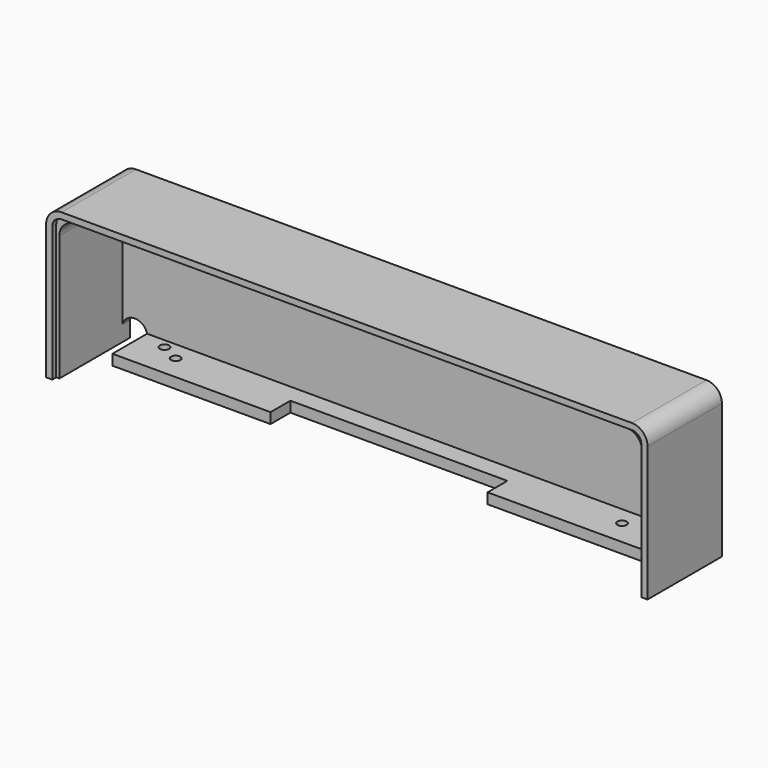
from build123d import *

# Parameters (mm, degrees)
F1_DEPTH = 30
F2_DEPTH = 28.4
F0_W     = 2.5
F0_H     = 3.4
F0_W_2   = 3
F0_W_3   = 7
F0_W_4   = 35.5
F0_W_5   = 70
F3_DEPTH = 17
F0_R     = 1.75
F4_DEPTH = 3
F6_DEPTH = 25
F7_R     = 1.5
F7_W     = 70
F7_H     = 13.8912867606
F8_DEPTH = 25


# Not quite as in the source:
# - ends of sketch curves that miss each other by under 0.0002 mm in the source are joined


with BuildPart() as f1:
    # F0 (on Front) → F1 (new body)
    with BuildSketch(Plane.XZ):
        with BuildLine():
            Line((-180.478038, -29.2658), (-180.478038, -72.7658))
            Line((-180.478038, -72.7658), (-178.478038, -72.7658))
            Line((-178.478038, -72.7658), (-178.478038, -29.2658))
            ThreePointArc((-178.478038, -29.2658), (-177.5993583436, -27.1444796564), (-175.478038, -26.2658))
            Line((-175.478038, -26.2658), (8.521962, -26.2658))
            ThreePointArc((8.521962, -26.2658), (10.6432823436, -27.1444796564), (11.521962, -29.2658))
            Line((11.521962, -29.2658), (11.521962, -71.1658))
            Line((11.521962, -71.1658), (11.521962, -72.7658))
            Line((11.521962, -72.7658), (13.521962, -72.7658))
            Line((13.521962, -72.7658), (13.521962, -29.2658))
            ThreePointArc((13.521962, -29.2658), (12.0574959059, -25.7302660941), (8.521962, -24.2658))
            Line((8.521962, -24.2658), (-175.478038, -24.2658))
            ThreePointArc((-175.478038, -24.2658), (-179.0135719059, -25.7302660941), (-180.478038, -29.2658))
        make_face()
    extrude(amount=F1_DEPTH)

    # F0 (on Front) → F2 (join)
    with BuildSketch(Plane.XZ):
        with BuildLine():
            Line((-178.478038, -29.2658), (-178.478038, -72.7658))
            Line((-178.478038, -72.7658), (-177.478038, -72.7658))
            Line((-177.478038, -72.7658), (-177.478038, -67.7658000352))
            Line((-177.478038, -67.7658000352), (-177.478038, -32.2658))
            ThreePointArc((-177.478038, -32.2658), (-176.0135719059, -28.7302660941), (-172.478038, -27.2658))
            Line((-172.478038, -27.2658), (5.521962, -27.2658))
            ThreePointArc((5.521962, -27.2658), (9.0574959059, -28.7302660941), (10.521962, -32.2658))
            Line((10.521962, -32.2658), (10.521962, -62.7658))
            Line((10.521962, -62.7658), (10.521962, -71.1658))
            Line((10.521962, -71.1658), (11.521962, -71.1658))
            Line((11.521962, -71.1658), (11.521962, -29.2658))
            ThreePointArc((11.521962, -29.2658), (10.6432823436, -27.1444796564), (8.521962, -26.2658))
            Line((8.521962, -26.2658), (-175.478038, -26.2658))
            ThreePointArc((-175.478038, -26.2658), (-177.5993583436, -27.1444796564), (-178.478038, -29.2658))
        make_face()
    extrude(amount=F2_DEPTH)

    # F0 (on Front) → F3 (join)
    with BuildSketch(Plane.XZ):
        with Locations((-168.228038, -69.4658)):
            Rectangle(F0_W, F0_H)
        with Locations((-165.478038, -69.4658)):
            Rectangle(F0_W_2, F0_H)
        with Locations((-160.478038, -69.4658)):
            Rectangle(F0_W_3, F0_H)
        with Locations((-155.478038, -69.4658)):
            Rectangle(F0_W_2, F0_H)
        with Locations((-136.228038, -69.4658)):
            Rectangle(F0_W_4, F0_H)
        with Locations((-83.478038, -69.4658)):
            Rectangle(F0_W_5, F0_H)
        with Locations((-30.728038, -69.4658)):
            Rectangle(F0_W_4, F0_H)
        with Locations((-11.478038, -69.4658)):
            Rectangle(F0_W_2, F0_H)
        with Locations((-6.478038, -69.4658)):
            Rectangle(F0_W_3, F0_H)
        with Locations((-1.478038, -69.4658)):
            Rectangle(F0_W_2, F0_H)
        with BuildLine():
            Line((0.021962, -71.1658), (10.521962, -71.1658))
            Line((10.521962, -71.1658), (10.521962, -62.7658))
            ThreePointArc((10.521962, -62.7658), (9.0574959059, -66.3013339059), (5.521962, -67.7658))
            Line((5.521962, -67.7658), (0.021962, -67.7658))
            Line((0.021962, -67.7658), (0.021962, -71.1658))
        make_face()
    extrude(amount=F3_DEPTH)

    # F0 (on Front) → F4 (join)
    with BuildSketch(Plane.XZ):
        Polygon((-166.978038, -71.1658), (-169.478038, -71.1658), (-169.478038, -72.7658), (11.521962, -72.7658), (11.521962, -71.1658), (10.521962, -71.1658), (0.021962, -71.1658), (-2.978038, -71.1658), (-9.978038, -71.1658), (-12.978038, -71.1658), (-48.478038, -71.1658), (-118.478038, -71.1658), (-153.978038, -71.1658), (-156.978038, -71.1658), (-163.978038, -71.1658), align=None)
        with BuildLine():
            Line((-177.478038, -32.2658), (-177.478038, -67.7658000352))
            ThreePointArc((-177.478038, -67.7658000352), (-173.478038, -64.726809), (-169.4780381264, -67.7658000352))
            Line((-169.4780381264, -67.7658000352), (-166.978038, -67.7658))
            Line((-166.978038, -67.7658), (-163.978038, -67.7658))
            Line((-163.978038, -67.7658), (-156.978038, -67.7658))
            Line((-156.978038, -67.7658), (-153.978038, -67.7658))
            Line((-153.978038, -67.7658), (-118.478038, -67.7658))
            Line((-118.478038, -67.7658), (-48.478038, -67.7658))
            Line((-48.478038, -67.7658), (-12.978038, -67.7658))
            Line((-12.978038, -67.7658), (-9.978038, -67.7658))
            Line((-9.978038, -67.7658), (-2.978038, -67.7658))
            Line((-2.978038, -67.7658), (0.021962, -67.7658))
            Line((0.021962, -67.7658), (5.521962, -67.7658))
            ThreePointArc((5.521962, -67.7658), (9.0574959059, -66.3013339059), (10.521962, -62.7658))
            Line((10.521962, -62.7658), (10.521962, -32.2658))
            ThreePointArc((10.521962, -32.2658), (9.0574959059, -28.7302660941), (5.521962, -27.2658))
            Line((5.521962, -27.2658), (-172.478038, -27.2658))
            ThreePointArc((-172.478038, -27.2658), (-176.0135719059, -28.7302660941), (-177.478038, -32.2658))
        make_face()
        with Locations((-66.878038, -40.4658)):
            Circle(F0_R, mode=Mode.SUBTRACT)
    extrude(amount=F4_DEPTH)

    # F7 (on offset) → F8 (cut)
    with BuildSketch(Plane.XY.offset(-75)):
        with Locations((-11.478038, -9)):
            Circle(F7_R)
        with Locations((-5.478038, -6)):
            Circle(F7_R)
        with Locations((-83.478038, -15.9456433803)):
            Rectangle(F7_W, F7_H)
        with Locations((-161.478038, -6)):
            Circle(F7_R)
        with Locations((-155.478038, -9)):
            Circle(F7_R)
    extrude(amount=F8_DEPTH, mode=Mode.SUBTRACT)


with BuildPart() as f6:
    # F0 (on Front) → F6 (new body)
    with BuildSketch(Plane.XZ):
        Polygon((-177.478038, 13.4356050125), (-177.478038, 12.671673), (-169.478038, 12.671673), (-169.478038, 27.071673), (-118.478038, 27.071673), (-118.478038, 19.571673), (-48.478038, 19.571673), (-48.478038, 27.071673), (10.521962, 27.071673), (10.521962, 38.071673), (-177.478038, 38.071673), (-177.478038, 33.071673), align=None)
    extrude(amount=F6_DEPTH)


solid = f1.part
